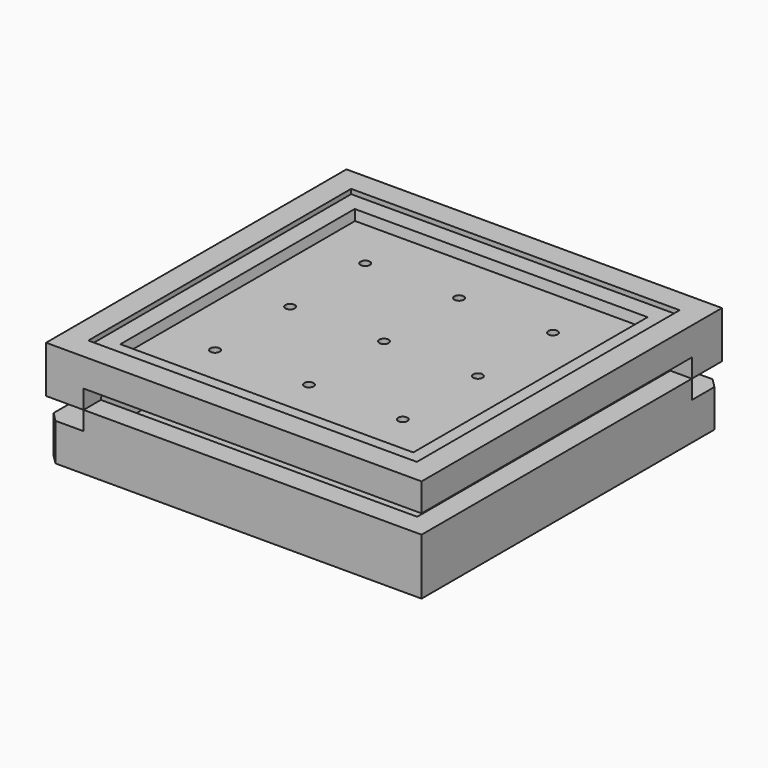
from build123d import *

# Parameters (mm, degrees)
F0_W      = 40
F0_H      = 40
F1_DEPTH  = 6
F4_W      = 40
F4_H      = 40
F5_DEPTH  = 3
F2_W      = 35.4
F2_H      = 35.4
F6_DEPTH  = 4
F6_TAPER  = 10
F8_W      = 35.4
F8_H      = 35.4
F9_DEPTH  = 1
F9_TAPER  = 10
F10_T     = -2.5
F11_R     = 0.5
F12_DEPTH = 2.5
F12_TAPER = -5
F13_SIZE  = 1
F14_W     = 4
F14_H     = 4
F15_DEPTH = 2
F17_W     = 4
F17_H     = 4
F18_DEPTH = 2
F19_W     = 35.0473460386
F19_H     = 35.0473460386
F20_DEPTH = 25
F20_TAPER = -10


with BuildPart() as f1:
    # F0 (on Top) → F1 (new body)
    with BuildSketch(Plane.XY):
        with Locations((20, 20)):
            Rectangle(F0_W, F0_H)
    extrude(amount=F1_DEPTH)

    # F2 (on face) → F6 (cut)
    with BuildSketch(Plane.XY.offset(6)):
        with Locations((20, 20)):
            Rectangle(F2_W, F2_H)
    extrude(amount=-F6_DEPTH, taper=F6_TAPER, mode=Mode.SUBTRACT)

    # F13
    f13_edges = [f1.edges().sort_by_distance(p)[0] for p in [
        (0, 0, 3),
        (40, 40, 3),
    ]]
    chamfer(f13_edges, length=F13_SIZE)

    # F14 (on face) → F15 (cut)
    with BuildSketch(Plane.XY.offset(6)):
        with Locations((2, 2)):
            Rectangle(F14_W, F14_H)
        with Locations((38, 38)):
            Rectangle(F14_W, F14_H)
    extrude(amount=-F15_DEPTH, mode=Mode.SUBTRACT)


with BuildPart() as f5:
    # F4 (on offset) → F5 (new body)
    with BuildSketch(Plane.XY.offset(11)):
        with Locations((20, 20)):
            Rectangle(F4_W, F4_H)
    extrude(amount=-F5_DEPTH)

    # F8 (on face) → F9 (join)
    with BuildSketch(Plane(origin=(0, 0, 8), x_dir=(1, 0, 0), z_dir=(0, 0, -1))):
        with Locations((20, -20)):
            Rectangle(F8_W, F8_H)
    extrude(amount=F9_DEPTH, taper=F9_TAPER)

    # F10
    f10_openings = [f5.faces().sort_by_distance(p)[0] for p in [
        (20, 20, 11),
    ]]
    offset(amount=F10_T, openings=f10_openings, kind=Kind.INTERSECTION)

    # F11 (on face) → F12 (cut, through all)
    with BuildSketch(Plane.XY.offset(9.5)):
        with Locations((10, 30)):
            Circle(F11_R)
        with Locations((20, 30)):
            Circle(F11_R)
        with Locations((30, 30)):
            Circle(F11_R)
        with Locations((10, 20)):
            Circle(F11_R)
        with Locations((10, 10)):
            Circle(F11_R)
        with Locations((20, 20)):
            Circle(F11_R)
        with Locations((20, 10)):
            Circle(F11_R)
        with Locations((30, 20)):
            Circle(F11_R)
        with Locations((30, 10)):
            Circle(F11_R)
    extrude(amount=-F12_DEPTH, taper=F12_TAPER, mode=Mode.SUBTRACT)

    # F17 (on face) → F18 (join)
    with BuildSketch(Plane(origin=(0, 0, 8), x_dir=(1, 0, 0), z_dir=(0, 0, -1))):
        with Locations((2, -2)):
            Rectangle(F17_W, F17_H)
        with Locations((38, -38)):
            Rectangle(F17_W, F17_H)
    extrude(amount=F18_DEPTH)

    # F19 (on face) → F20 (cut)
    with BuildSketch(Plane(origin=(0, 0, 7), x_dir=(1, 0, 0), z_dir=(0, 0, -1))):
        with Locations((20, -20)):
            Rectangle(F19_W, F19_H)
    extrude(amount=F20_DEPTH, taper=F20_TAPER, mode=Mode.SUBTRACT)


solid = Compound([f1.part, f5.part])
